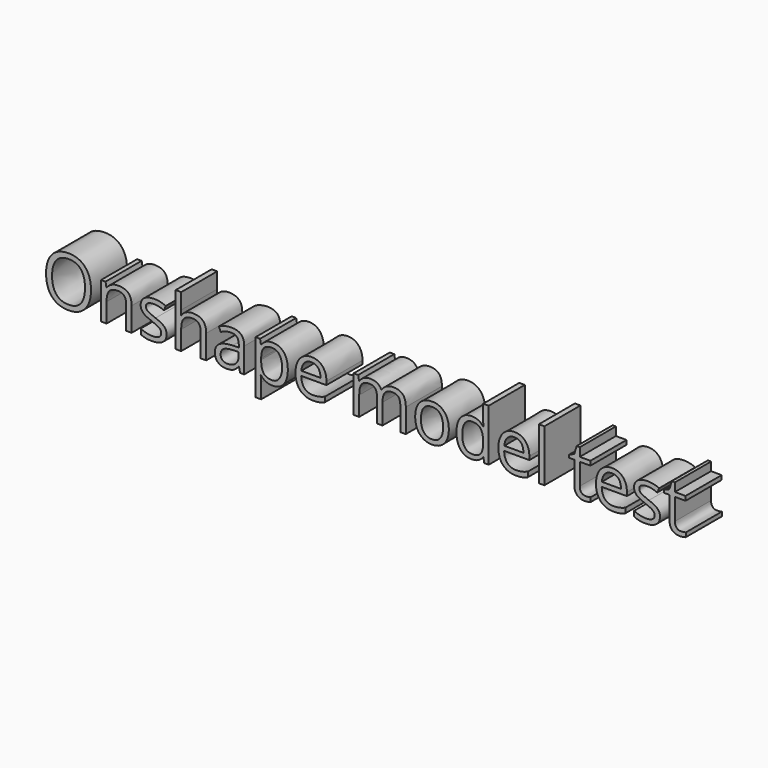
from build123d import *

# Parameters (mm, degrees)
F0_TEXT_SIZE = 37.8885823819
F1_DEPTH     = 25


# Not quite as in the source:
# - Text() gives the source's letters only with a copy of the font that has no kerning and outlines rounded to 1/6400 em; it was checked with that copy


with BuildPart() as f1:
    # F0 (on Front) → F1 (new body)
    with BuildSketch(Plane.XZ):
        with Locations((0, 0)):
            Text('Onshape model test', F0_TEXT_SIZE, font='Open Sans', text_align=(TextAlign.LEFT, TextAlign.BOTTOM))
    extrude(amount=F1_DEPTH)


solid = f1.part
